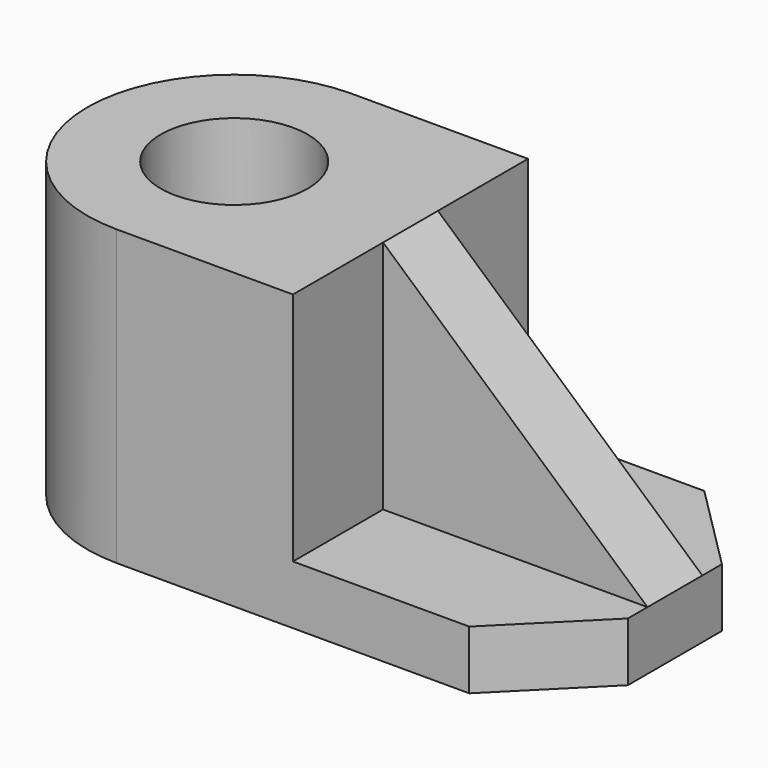
from build123d import *

# Parameters (mm, degrees)
F0_W      = 60
F0_H      = 30
F1_DEPTH  = 30
F2_R      = 14.99999
F3_SIZE   = 9
F4_R      = 7.5
F5_DEPTH  = 30
F6_W      = 9
F6_H      = 24
F6_W_2    = 18
F7_DEPTH  = 11.5
F8_START  = -18.5
F6_W_3    = 27
F8_DEPTH  = 11.501
F10_DEPTH = 7


# Not quite as in the source:
# - a fillet or chamfer is up to 0.001 mm smaller than in the source, because OpenCascade refuses the exact size


with BuildPart() as f1:
    # F0 (on Top) → F1 (new body)
    with BuildSketch(Plane.XY):
        with Locations((0, 0.9866876062)):
            Rectangle(F0_W, F0_H)
    extrude(amount=F1_DEPTH)

    # F2 (radius 15 in the source; OpenCascade refuses exactly that, so slightly less here)
    f2_edges = [f1.edges().sort_by_distance(p)[0] for p in [
        (-30, -14.013312, 15),
        (-30, 15.986688, 15),
    ]]
    fillet(f2_edges, radius=F2_R)

    # F3
    f3_edges = [f1.edges().sort_by_distance(p)[0] for p in [
        (30, -14.013312, 15),
        (30, 15.986688, 15),
    ]]
    chamfer(f3_edges, length=F3_SIZE)

    # F4 (on face) → F5 (cut, through all)
    with BuildSketch(Plane.XY.offset(30)):
        with Locations((-15, 0.9866876062)):
            Circle(F4_R)
    extrude(amount=-F5_DEPTH, mode=Mode.SUBTRACT)

    # F6 (on face) → F7 (cut)
    with BuildSketch(Plane.XZ.offset(14.0133123938)):
        with Locations((25.5, 18)):
            Rectangle(F6_W, F6_H)
        with Locations((12, 18)):
            Rectangle(F6_W_2, F6_H)
    extrude(amount=-F7_DEPTH, mode=Mode.SUBTRACT)

    # F6 (on face) → F8 (cut)
    with BuildSketch(Plane.XZ.offset(14.0133123938).offset(F8_START)):
        with Locations((16.5, 18)):
            Rectangle(F6_W_3, F6_H)
    extrude(amount=-F8_DEPTH, mode=Mode.SUBTRACT)

    # F9 (on face) → F10 (cut, through all)
    with BuildSketch(Plane.XZ.offset(2.5133123938)):
        Polygon((3, 30), (30, 6), (30, 30), align=None)
    extrude(amount=-F10_DEPTH, mode=Mode.SUBTRACT)


solid = f1.part
